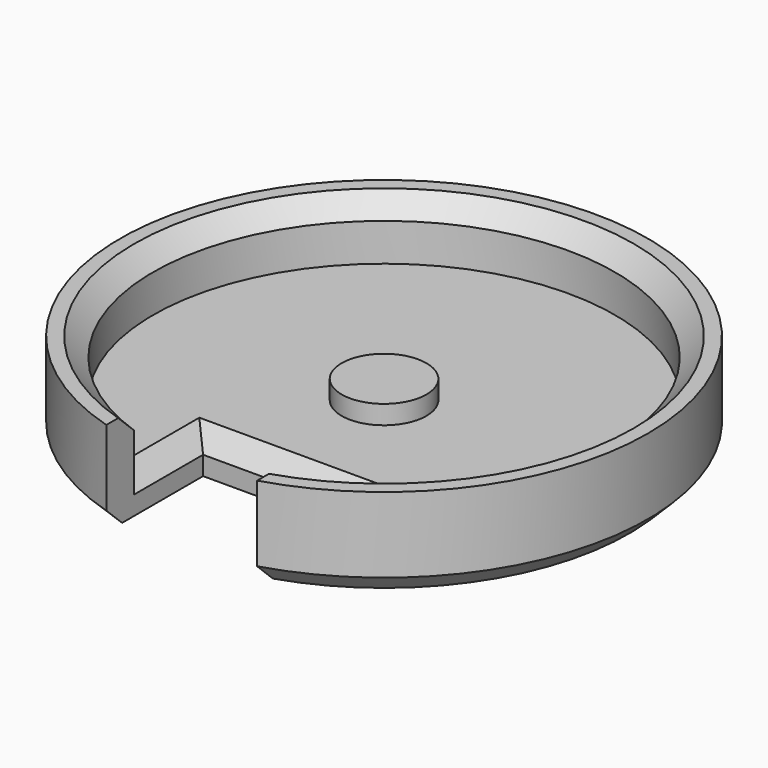
from build123d import *

# Parameters (mm, degrees)
F0_R     = 2.25
F1_DEPTH = 2
F2_DEPTH = 5
F3_DEPTH = 3
F4_SIZE  = 0.99999


# Not quite as in the source:
# - a fillet or chamfer is up to 0.001 mm smaller than in the source, because OpenCascade refuses the exact size


with BuildPart() as f1:
    # F0 (on Top) → F1 (new body)
    with BuildSketch(Plane.XY):
        with BuildLine():
            ThreePointArc((4, -13.416407865), (11.2249721603, -8.3666002653), (14, 0))
            ThreePointArc((14, 0), (-8.3666002653, 11.2249721603), (-4, -13.416407865))
            Line((-4, -13.416407865), (-4, -11.5785361769))
            ThreePointArc((-4, -11.5785361769), (-7.1085336041, 9.9765349696), (12.25, 0))
            ThreePointArc((12.25, 0), (9.9765349696, -7.1085336041), (4, -11.5785361769))
            Line((4, -11.5785361769), (4, -13.416407865))
        make_face()
        with BuildLine():
            ThreePointArc((12.25, 0), (-7.1085336041, 9.9765349696), (-4, -11.5785361769))
            Line((-4, -11.5785361769), (-4, -7))
            Line((-4, -7), (4, -7))
            Line((4, -7), (4, -11.5785361769))
            ThreePointArc((4, -11.5785361769), (9.9765349696, -7.1085336041), (12.25, 0))
        make_face()
        Circle(F0_R, mode=Mode.SUBTRACT)
        Circle(F0_R)
    extrude(amount=F1_DEPTH)

    # F0 (on Top) → F2 (join)
    with BuildSketch(Plane.XY):
        with BuildLine():
            ThreePointArc((4, -13.416407865), (11.2249721603, -8.3666002653), (14, 0))
            ThreePointArc((14, 0), (-8.3666002653, 11.2249721603), (-4, -13.416407865))
            Line((-4, -13.416407865), (-4, -11.5785361769))
            ThreePointArc((-4, -11.5785361769), (-7.1085336041, 9.9765349696), (12.25, 0))
            ThreePointArc((12.25, 0), (9.9765349696, -7.1085336041), (4, -11.5785361769))
            Line((4, -11.5785361769), (4, -13.416407865))
        make_face()
    extrude(amount=F2_DEPTH)

    # F0 (on Top) → F3 (join)
    with BuildSketch(Plane.XY):
        Circle(F0_R)
    extrude(amount=F3_DEPTH)

    # F4 (size 1 in the source; OpenCascade refuses exactly that, so slightly less here)
    f4_edges = [f1.edges().sort_by_distance(p)[0] for p in [
        (0, 14, 0),
        (-7.108534, 9.976535, 5),
        (0, -7, 2),
        (-4, -9.289268, 2),
        (4, -9.289268, 2),
    ]]
    chamfer(f4_edges, length=F4_SIZE)


solid = f1.part
